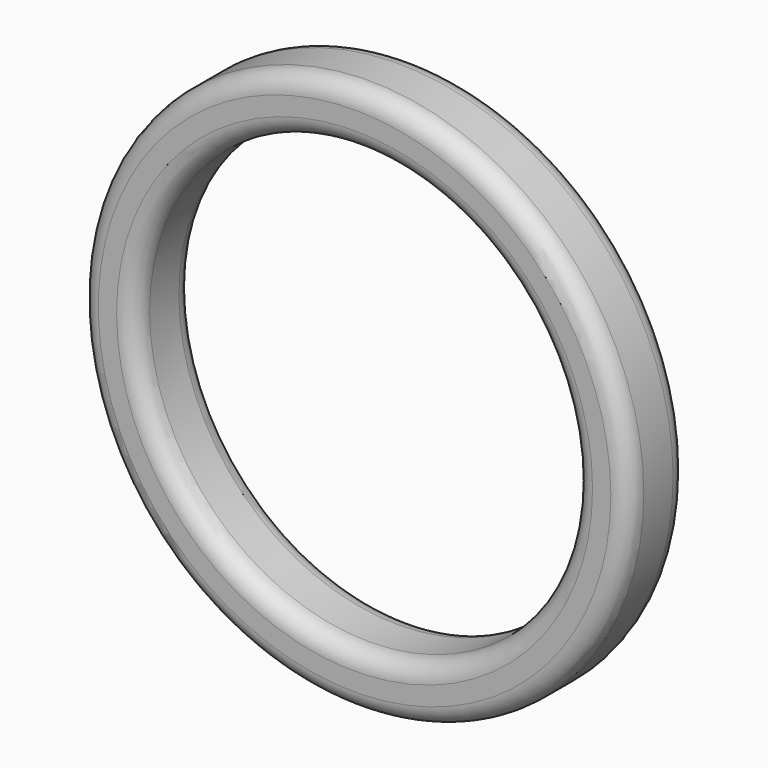
from build123d import *

# Parameters (mm, degrees)
F0_R     = 7.5
F0_R_2   = 6
F1_DEPTH = 2
F2_R     = 0.5


# Not quite as in the source:
# - the program builds the solid bodies; features that only make, move or delete a surface that nothing else refers to are left out


with BuildPart() as f1:
    # F0 (on Front) → F1 (new body)
    with BuildSketch(Plane.XZ):
        with Locations((0, 92.6766253437)):
            Circle(F0_R)
        with Locations((0, 92.6766253437)):
            Circle(F0_R_2, mode=Mode.SUBTRACT)
    extrude(amount=F1_DEPTH)

    # F2
    f2_edges = [f1.edges().sort_by_distance(p)[0] for p in [
        (-7.5, -2, 92.676625),
        (-6, -2, 92.676625),
        (-7.5, 0, 92.676625),
        (-6, 0, 92.676625),
    ]]
    fillet(f2_edges, radius=F2_R)


solid = f1.part
